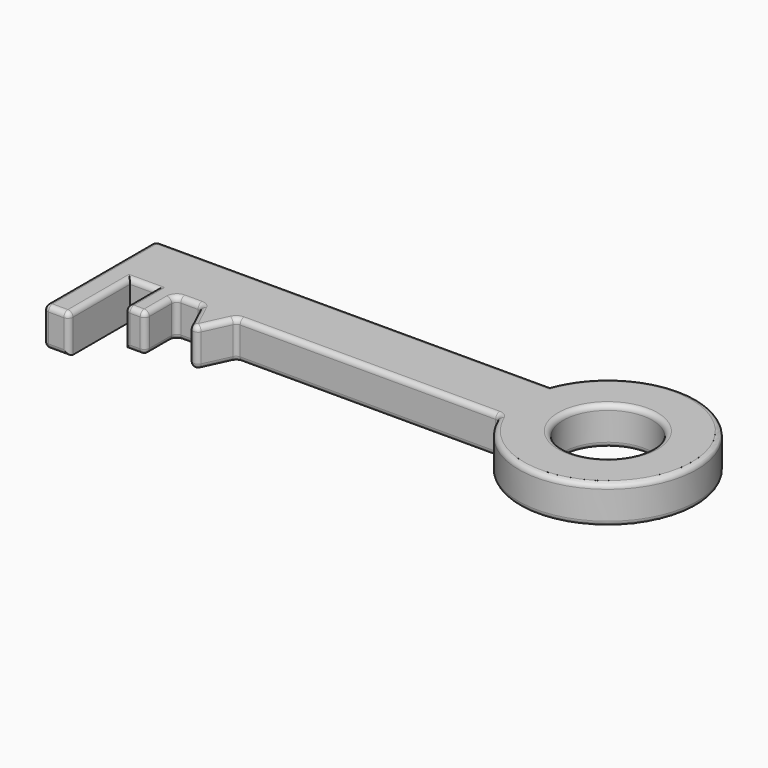
from build123d import *

# Parameters (mm, degrees)
F0_W     = 8
F0_H     = 15
F0_W_2   = 10
F0_H_2   = 30
F0_R     = 17.5
F1_DEPTH = 15
F2_R     = 2


with BuildPart() as f1:
    # F0 (on Top) → F1 (new body)
    with BuildSketch(Plane.XY):
        Polygon((-113.2757292581, 0), (-106.275600045, 15), (-120.275600045, 15), align=None)
        with Locations((-134.275600045, 7.5)):
            Rectangle(F0_W, F0_H)
        with Locations((-153.275600045, 0)):
            Rectangle(F0_W_2, F0_H_2)
        with BuildLine():
            Line((-3.275600045, 40), (-158.275600045, 40))
            Line((-158.275600045, 40), (-158.275600045, 15))
            Line((-158.275600045, 15), (-148.275600045, 15))
            Line((-148.275600045, 15), (-138.275600045, 15))
            Line((-138.275600045, 15), (-130.275600045, 15))
            Line((-130.275600045, 15), (-120.275600045, 15))
            Line((-120.275600045, 15), (-106.275600045, 15))
            Line((-106.275600045, 15), (-3.275600045, 15))
            ThreePointArc((-3.275600045, 15), (64.4161420316, 27.5), (-3.275600045, 40))
        make_face()
        with Locations((29.4161420316, 27.5)):
            Circle(F0_R, mode=Mode.SUBTRACT)
    extrude(amount=F1_DEPTH)

    # F2
    f2_edges = [f1.edges().sort_by_distance(p)[0] for p in [
        (-80.7756, 40, 15),
        (-54.7756, 15, 15),
        (-116.775665, 7.5, 15),
        (-109.775665, 7.5, 15),
        (-130.2756, 7.5, 15),
        (-134.2756, 0, 15),
        (-143.2756, 15, 15),
        (-138.2756, 7.5, 15),
        (-148.2756, 0, 15),
        (-153.2756, -15, 15),
        (-158.2756, 12.5, 15),
        (64.416142, 27.5, 15),
        (11.916142, 27.5, 15),
        (-106.2756, 15, 7.5),
        (-3.2756, 15, 7.5),
        (-54.7756, 15, 0),
        (-109.775665, 7.5, 0),
        (-113.275729, 0, 7.5),
        (-116.775665, 7.5, 0),
        (-120.2756, 15, 7.5),
        (-134.2756, 0, 0),
        (-130.2756, 0, 7.5),
        (-138.2756, 0, 7.5),
        (-158.2756, -15, 7.5),
        (-148.2756, -15, 7.5),
        (-153.2756, -15, 0),
        (-158.2756, 40, 7.5),
        (-158.2756, 12.5, 0),
        (-80.7756, 40, 0),
        (64.416142, 27.5, 0),
        (46.916142, 27.5, 7.5),
        (11.916142, 27.5, 0),
        (-125.2756, 15, 0),
        (-130.2756, 15, 7.5),
        (-125.2756, 15, 15),
        (-130.2756, 7.5, 0),
    ]]
    fillet(f2_edges, radius=F2_R)


solid = f1.part
